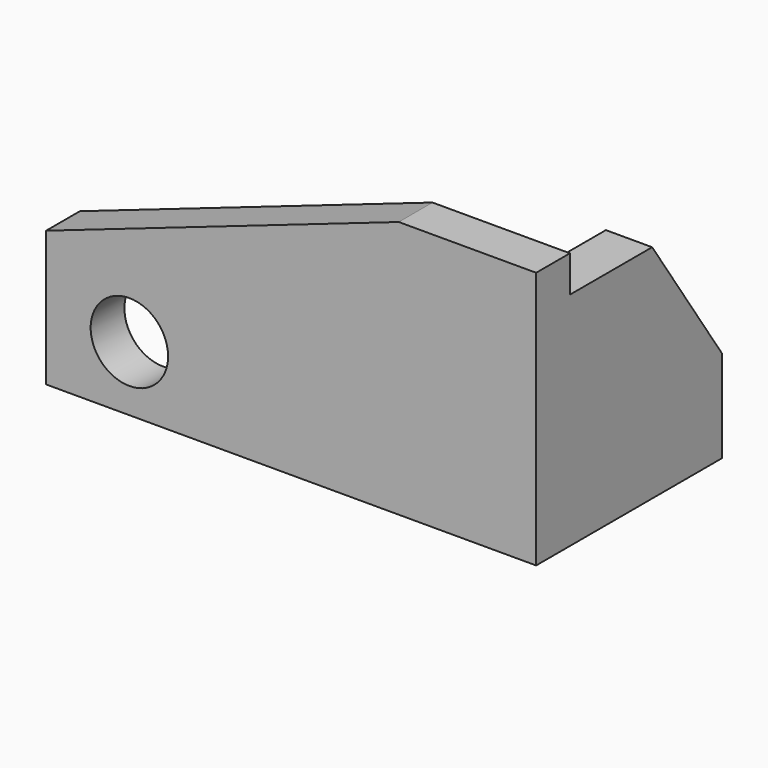
from build123d import *

# Parameters (mm, degrees)
F0_W        = 19.1829744726
F0_H        = 41.2798188627
F1_DEPTH    = 8.636
F2_W        = 65.804887563
F2_H        = 25.253537111
F2_R        = 7.2247324081
F3_DEPTH    = 7.874
F4_W        = 40.3897017241
F4_H        = 12.0197124779
F5_DEPTH    = 25.4
F6_T4_DEPTH = 221.0461057398


# Not quite as in the source:
# - a fillet or chamfer that OpenCascade refuses, or shapes differently, is made with other operations: its cross-section is extruded or revolved along the edge and cut away or added


with BuildPart() as f1:
    # F0 (on Right) → F1 (new body)
    with BuildSketch(Plane.YZ):
        with Locations((9.5914872363, 8.6201969534)):
            Rectangle(F0_W, F0_H)
        Polygon((35.4520790279, 5.2206832916), (19.1829744726, 29.2601063848), (19.1829744726, -12.0197124779), (35.4520790279, -12.0197124779), align=None)
    extrude(amount=F1_DEPTH)

    # F2 (on face) → F3 (join)
    with BuildSketch(Plane.XZ):
        Polygon((-16.9975720346, -12.0197124779), (8.636, -12.0197124779), (8.636, 36.0591337085), (-16.9975720346, 36.0591337085), (-16.9975720346, 13.2338246331), align=None)
        with Locations((-49.9000158161, 0.6070560776)):
            Rectangle(F2_W, F2_H)
        with Locations((-67.2618225217, 0)):
            Circle(F2_R, mode=Mode.SUBTRACT)
        Polygon((-82.8024595976, 13.2338246331), (-16.9975720346, 13.2338246331), (-16.9975720346, 36.0591337085), align=None)
    extrude(amount=F3_DEPTH)

    # F4 (on face) → F5 (join)
    with BuildSketch(Plane(origin=(0, 0, 0), x_dir=(-1, 0, 0), z_dir=(0, 1, 0))):
        with Locations((20.194850862, -6.009856239)):
            Rectangle(F4_W, F4_H)
    extrude(amount=F5_DEPTH)

    # F6: chamfer of 40.64 on 1 edges, made by hand


with BuildPart() as f6_tool2:
    # F6_s3 → F6_t4 (new body)
    with BuildSketch(Plane.XY.offset(-116.5329091089)):
        Polygon((-40.3897017241, -15.24), (0.2502982759, 25.4), (-40.3897017241, 25.4), align=None)
    extrude(amount=F6_T4_DEPTH)

    split(bisect_by=Plane.XZ, keep=Keep.BOTTOM)

    split(bisect_by=Plane.YZ, keep=Keep.BOTTOM)


with BuildPart() as f1_1:
    add(f1.part)

    # F6_t1: cut F6_tool2
    add(f6_tool2.part, mode=Mode.SUBTRACT)


solid = f1_1.part
